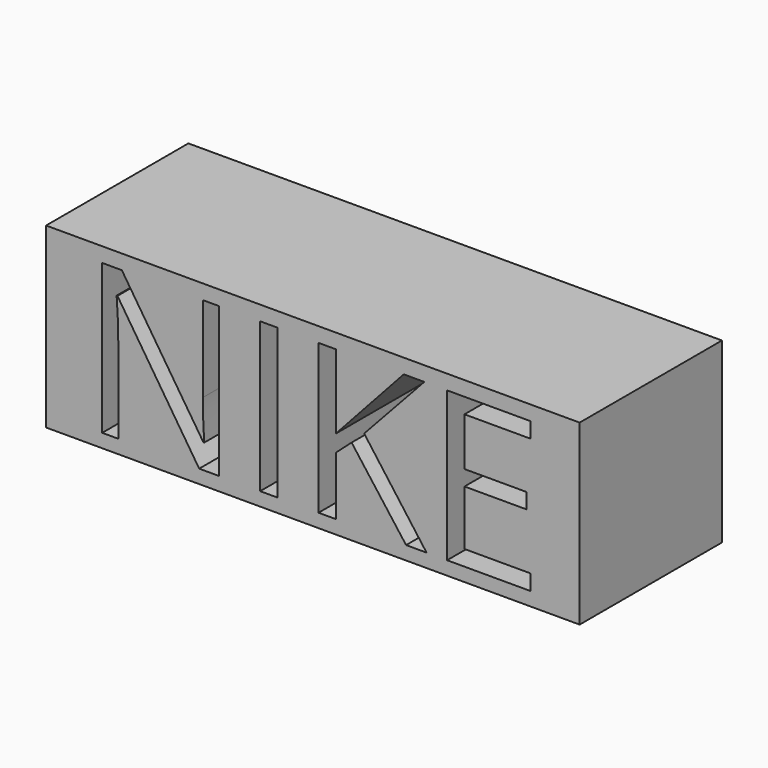
from build123d import *

# Parameters (mm, degrees)
F0_W         = 76.2
F0_H         = 50.8
F1_DEPTH     = 25.4
F2_TEXT_SIZE = 29.9183124513
F3_DEPTH     = 25.4
F4_W         = 76.2
F4_H         = 25.4
F5_DEPTH     = 25.4


# Not quite as in the source:
# - Text() gives the source's letters only with a copy of the font that has no kerning and outlines rounded to 1/6400 em; it was checked with that copy


with BuildPart() as f1:
    # F0 (on Front) → F1 (new body)
    with BuildSketch(Plane.XZ):
        with Locations((38.1, 25.4)):
            Rectangle(F0_W, F0_H)
    extrude(amount=F1_DEPTH)

    # F2 (on face) → F3 (cut)
    with BuildSketch(Plane.XZ.offset(25.4)):
        with Locations((5.08, 1.941276721)):
            Text('NIKE', F2_TEXT_SIZE, font='Open Sans', text_align=(TextAlign.LEFT, TextAlign.BOTTOM))
    extrude(amount=-F3_DEPTH, mode=Mode.SUBTRACT)

    # F4 (on face) → F5 (cut)
    with BuildSketch(Plane.XZ.offset(25.4)):
        with Locations((38.1, 38.1)):
            Rectangle(F4_W, F4_H)
    extrude(amount=-F5_DEPTH, mode=Mode.SUBTRACT)


solid = f1.part
